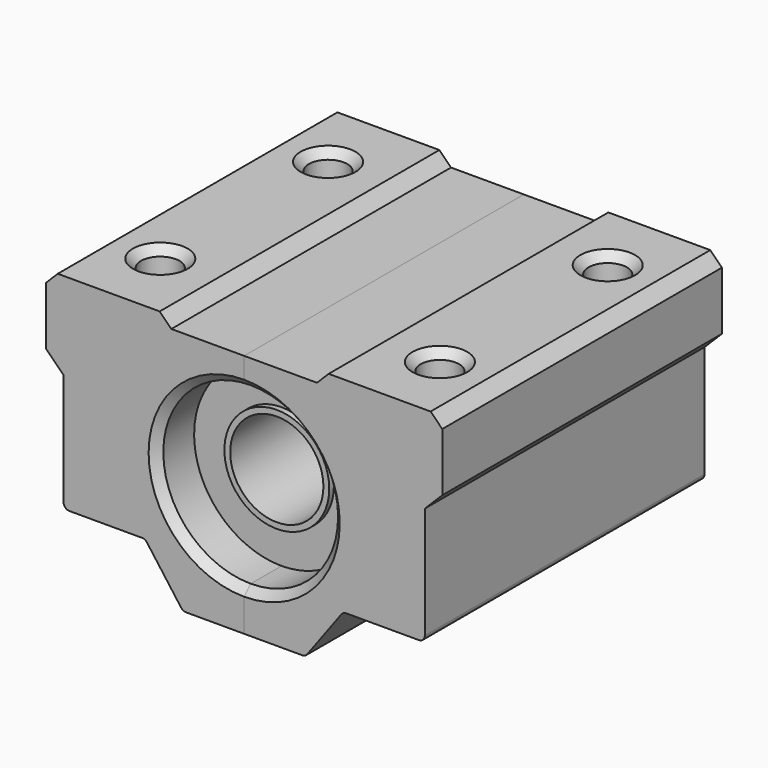
from build123d import *
from build123d import SkipClean  # not in build123d's __all__

# Parameters (mm, degrees)
F1_DEPTH       = 15
F2_SIZE        = 0.99999
F3_SIZE        = 1.49999
F4_R           = 0.5
F6_D           = 3
F6_CBORE_D     = 3.3
F6_CBORE_DEPTH = 6
F7_SIZE        = 0.7
F0_R           = 4.5
F8_DEPTH       = 11
F0_R_2         = 4
F9_DEPTH       = 11.5


# Not quite as in the source:
# - a fillet or chamfer is up to 0.001 mm smaller than in the source, because OpenCascade refuses the exact size


with BuildPart() as f1:
    # F0 (on Front) → F1 (new body, symmetric)
    with BuildSketch(Plane.XZ):
        with BuildLine():
            ThreePointArc((0, 7.5), (5.3033008589, 5.3033008589), (7.5, 0))
            ThreePointArc((7.5, 0), (5.3033008589, -5.3033008589), (0, -7.5))
            Line((0, -7.5), (0, -11))
            Line((0, -11), (5.25, -11))
            Line((5.25, -11), (8.5, -6.6))
            Line((8.5, -6.6), (15.5, -6.6))
            Line((15.5, -6.6), (15.5, 3.5))
            Line((15.5, 3.5), (17, 3.5))
            Line((17, 3.5), (17, 11))
            Line((17, 11), (7.25, 11))
            Line((7.25, 11), (7.25, 10))
            Line((7.25, 10), (0, 10))
            Line((0, 10), (0, 7.5))
        make_face()
    extrude(amount=F1_DEPTH, both=True)

    # F2 (size 1 in the source; OpenCascade refuses exactly that, so slightly less here)
    f2_edges = [f1.edges().sort_by_distance(p)[0] for p in [
        (7.25, 0, 10),
        (17, 0, 11),
    ]]
    chamfer(f2_edges, length=F2_SIZE)

    # F3 (size 1.5 in the source; OpenCascade refuses exactly that, so slightly less here)
    f3_edges = [f1.edges().sort_by_distance(p)[0] for p in [
        (17, 0, 3.5),
    ]]
    chamfer(f3_edges, length=F3_SIZE)

    # F4
    f4_edges = [f1.edges().sort_by_distance(p)[0] for p in [
        (15.5, 0, -6.6),
        (8.5, 0, -6.6),
        (5.25, 0, -11),
    ]]
    fillet(f4_edges, radius=F4_R)

    # F6 (through all)
    with Locations(Plane.XY.offset(11)):
        with Locations((12, 9), (12, -9)):
            CounterBoreHole(F6_D / 2, F6_CBORE_D / 2, F6_CBORE_DEPTH)

    # F7
    f7_edges = [f1.edges().sort_by_distance(p)[0] for p in [
        (7.5, -15, 0),
        (7.5, 15, 0),
        (10.35, 9, 11),
        (10.35, -9, 11),
    ]]
    chamfer(f7_edges, length=F7_SIZE)

    # F10: F1 across plane


with BuildPart() as f8:
    # F0 (on Front) → F8 (new body, symmetric)
    with BuildSketch(Plane.XZ):
        with BuildLine():
            ThreePointArc((0, -7.5), (5.3033008589, -5.3033008589), (7.5, 0))
            ThreePointArc((7.5, 0), (5.3033008589, 5.3033008589), (0, 7.5))
            ThreePointArc((0, 7.5), (-7.5, 0), (0, -7.5))
        make_face()
        Circle(F0_R, mode=Mode.SUBTRACT)
    extrude(amount=F8_DEPTH, both=True)

    # F0 (on Front) → F9 (join, symmetric)
    with BuildSketch(Plane.XZ):
        Circle(F0_R)
        Circle(F0_R_2, mode=Mode.SUBTRACT)
    extrude(amount=F9_DEPTH, both=True)


with BuildPart() as f1_1:
    add(f1.part, clean=False)
    with SkipClean():  # cleaning this boolean's faces spoils the solid; the shape is the same uncleaned
        add(f1.part.mirror(Plane.YZ), clean=False)


solid = Compound([f8.part, f1_1.part])
